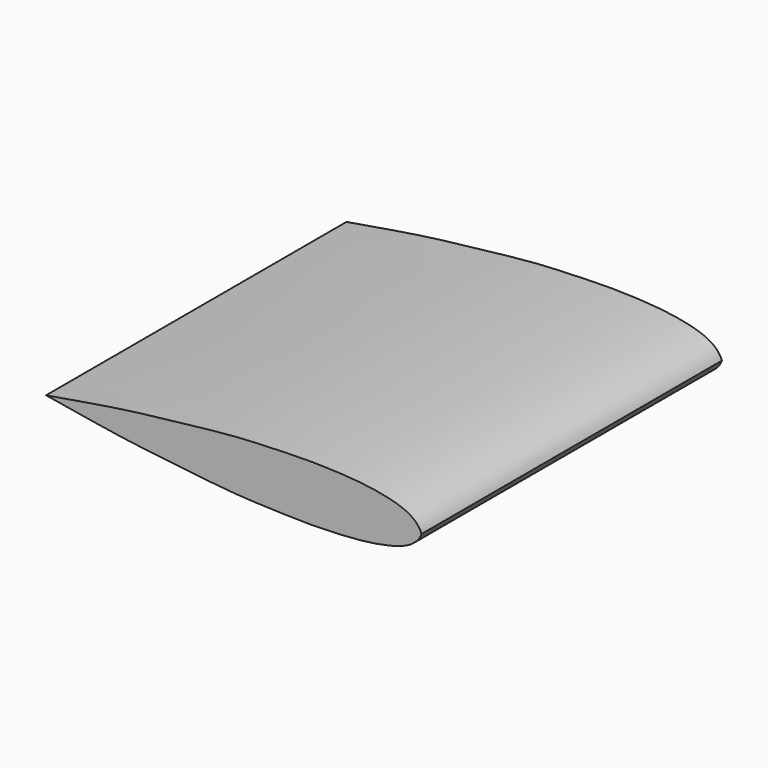
from build123d import *

# Parameters (mm, degrees)
F1_DEPTH = 1000


# Not quite as in the source:
# - the dataset's text gives a spline's control points without its knots; the knots are read off the source's solid


with BuildPart() as f1:
    # F0 (on Front) → F1 (new body)
    with BuildSketch(Plane.XZ):
        with BuildLine():
            add(Edge.make_bspline(
                [(500, -115.648996), (486.977463, -151.941312), (400.801148, -177.57307), (301.654339, -187.354019), (199.931158, -190.978969), (100.114038, -187.233363), (-0.383, -183.5495), (-133.736619, -168.403006), (-300.896358, -150.494586), (-433.383511, -126.440453), (-500, -115.648996)],
                knots=[0, 0, 0, 0, 115.673972, 216.368282, 316.340511, 416.288467, 517.16163, 617.576707, 818.863746, 1021.318453, 1021.318453, 1021.318453, 1021.318453], degree=3))
            add(Edge.make_bspline(
                [(500, -115.648996), (486.977463, -79.356681), (400.801148, -53.724923), (301.654339, -43.943974), (199.931158, -40.319024), (100.114038, -44.06463), (-0.383, -47.748493), (-133.736619, -62.894987), (-300.896358, -80.803407), (-433.383511, -104.85754), (-500, -115.648996)],
                knots=[0, 0, 0, 0, 115.673972, 216.368282, 316.340511, 416.288467, 517.16163, 617.576707, 818.863746, 1021.318453, 1021.318453, 1021.318453, 1021.318453], degree=3))
        make_face()
    extrude(amount=-F1_DEPTH)


with BuildPart() as f1_1:
    # F2: moved
    add(f1.part.moved(Location((500, 0, 115.648996))))


solid = f1_1.part
